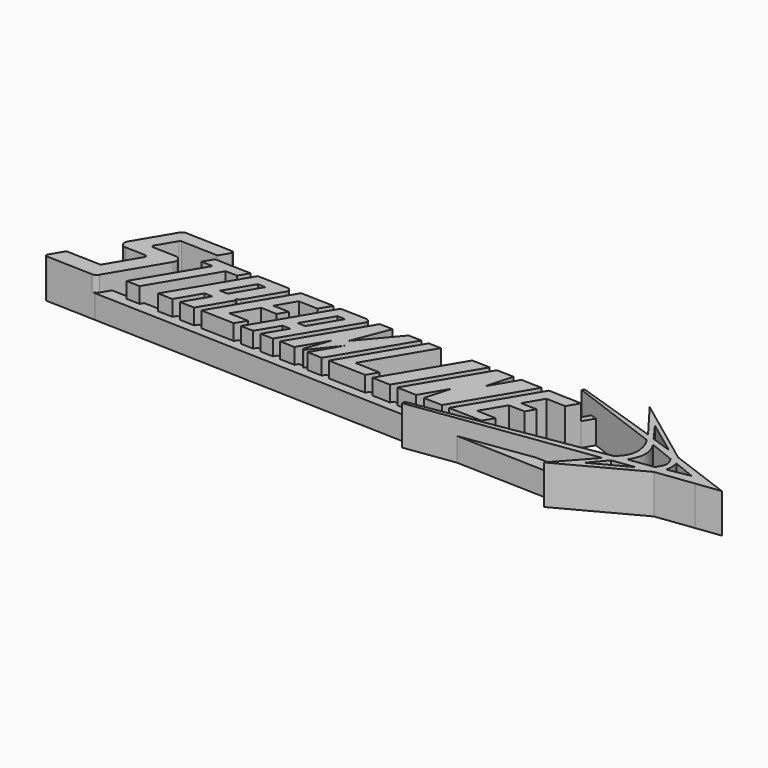
from build123d import *

# Parameters (mm, degrees)
F3_DEPTH    = 5
F4_DEPTH    = 3
F5_DEPTH    = 5
F6_T1_DEPTH = 4.2430941222
F7_R        = 0.75
F8_R        = 0.25
F9_R        = 0.5


# Not quite as in the source:
# - a fillet or chamfer that OpenCascade refuses, or shapes differently, is made with other operations: its cross-section is extruded or revolved along the edge and cut away or added
# - the dataset's text gives a spline's control points without its knots; the knots are read off the source's solid


with BuildPart() as f3:
    # F1 (on Top) → F3 (new body)
    with BuildSketch(Plane.XY):
        with BuildLine():
            Line((20.9890730849, 6.6955136709), (20.8262177718, 6.4128558685))
            Line((20.8262177718, 6.4128558685), (32.5976700121, 2.0520742269))
            add(Edge.make_bspline(
                [(32.5976700121, 2.0520742269), (32.66479791, 1.9612326634), (32.9078702036, 1.6322940043), (33.2495684632, 0.8503160257), (33.5175624456, -0.3144692674), (33.2543808955, -1.5649575024), (32.6660823722, -2.3242091008), (32.2798649798, -2.631161677), (32.1629690369, -2.724066847)],
                knots=[0, 0, 0, 0, 0.338377, 1.225264, 2.537513, 3.868989, 4.900887, 5.348773, 5.348773, 5.348773, 5.348773], degree=3))
            Line((32.1629690369, -2.724066847), (8.6369270261, -6.5884035475))
            Line((8.6369270261, -6.5884035475), (8.6392750964, -6.9738253951))
            Line((8.6392750964, -6.9738253951), (31.5857229554, -3.7504750461))
            Line((31.5857229554, -3.7504750461), (27.6476915727, -8.1477057948))
            Line((27.6476915727, -8.1477057948), (37.4754122714, -2.8992304066))
            Line((37.4754122714, -2.8992304066), (42.2447667452, -2.2940801703))
            Line((42.2447667452, -2.2940801703), (45.3573419295, -1.8991471414))
            Line((45.3573419295, -1.8991471414), (42.1900098482, -0.7209429398))
            Line((42.1900098482, -0.7209429398), (37.4064079021, 1.0584915391))
            Line((37.4064079021, 1.0584915391), (28.4184888939, 7.7636854948))
            Line((28.4184888939, 7.7636854948), (31.9932630947, 3.0268066577))
            Line((31.9932630947, 3.0268066577), (20.9890730849, 6.6955136709))
        make_face()
        Polygon((35.4575661162, -3.2228435634), (30.8492315292, -5.6525000589), (32.5873011966, -3.610950146), align=None, mode=Mode.SUBTRACT)
        with BuildLine():
            Line((36.9164326126, -2.0131677576), (33.7172948492, -2.4477515814))
            add(Edge.make_bspline(
                [(33.7522917412, 1.6292004342), (33.8151917165, 1.5224178068), (34.0236807852, 1.1684709092), (34.316701025, 0.4779029509), (34.496667936, -0.4792529836), (34.2653350207, -1.3976559433), (33.9756190313, -2.0377855614), (33.7761823537, -2.3542949446), (33.7172948492, -2.4477515814)],
                knots=[0, 0, 0, 0, 0.371596, 1.231709, 2.243752, 3.225396, 4.015779, 4.346939, 4.346939, 4.346939, 4.346939], degree=3))
            Line((33.7522917412, 1.6292004342), (37.0218462303, 0.3297472202))
            add(Edge.make_bspline(
                [(36.9164326126, -2.0131677576), (36.9641091848, -1.9397738205), (37.1152370901, -1.7071284219), (37.3297565887, -1.2919332808), (37.4856453978, -0.739306923), (37.33186312, -0.2383098734), (37.1684320619, 0.1026463975), (37.0557106146, 0.2772826387), (37.0218462303, 0.3297472202)],
                knots=[0, 0, 0, 0, 0.262319, 0.831507, 1.406816, 1.920771, 2.356545, 2.543685, 2.543685, 2.543685, 2.543685], degree=3))
        make_face(mode=Mode.SUBTRACT)
        with BuildLine():
            add(Edge.make_bspline(
                [(38.1416125443, -1.7388595712), (38.1499505224, -1.6861617751), (38.1779707155, -1.5090687116), (38.2120498589, -1.1831309562), (38.2229188343, -0.7827452769), (38.1747484177, -0.4294012981), (38.1198989231, -0.1979742905), (38.0817402166, -0.0923088934), (38.0715592092, -0.0641174199)],
                knots=[0, 0, 0, 0, 0.160044, 0.537838, 0.982775, 1.357504, 1.604535, 1.694427, 1.694427, 1.694427, 1.694427], degree=3))
            Line((38.0715592092, -0.0641174199), (40.9662755038, -1.2324347209))
            Line((40.9662755038, -1.2324347209), (38.1416125443, -1.7388595712))
        make_face(mode=Mode.SUBTRACT)
        Polygon((33.0280173393, 2.632852847), (31.3381946618, 4.9499999378), (35.6817278033, 1.7299066189), align=None, mode=Mode.SUBTRACT)
    extrude(amount=F3_DEPTH)

    # F2 (on Top) → F4 (join)
    with BuildSketch(Plane.XY):
        Polygon((30.4451698308, -5.0240238787), (-31.5077020799, -3.0337495602), (-32.4236048399, -4.5718295186), (29.0806183264, -6.5476907188), align=None)
        Polygon((21.6650361648, 4.1573069305), (22.5942029424, 4.1285426611), (23.3891042563, 5.4634243028), (22.6138332811, 5.7506265415), align=None)
    extrude(amount=F4_DEPTH)

    # F0 (on Top) → F5 (join)
    with BuildSketch(Plane.XY):
        Polygon((-37.9180402346, -2.274961737), (-39.1569778781, -4.3555157462), (-32.4236048399, -4.5718295186), (-27.5283611438, 3.6487770236), (-32.0936571446, 3.7954399806), (-30.4533826172, 6.5499609703), (-25.6068335268, 6.4052671518), (-24.6373546626, 8.0333177225), (-31.447669093, 8.2521032848), (-35.1129866215, 2.0969177364), (-30.8469119008, 1.959867448), (-33.4540838572, -2.4183690959), align=None)
        Polygon((-24.5548592656, 4.3197505292), (-29.241506667, -3.5505592413), (-27.5305965593, -3.603523984), (-22.8439491578, 4.2667857865), (-21.3778178633, 4.2213986756), (-20.6361838773, 5.4668282346), (-25.2816460752, 5.6106380753), (-26.0232800612, 4.3652085163), align=None)
        Polygon((-19.6843868267, 5.4373633985), (-25.1126682142, -3.678375931), (-23.2585706727, -3.7357733353), (-21.4998541289, -0.7823520914), (-20.5003329545, -0.813294326), (-22.2590494983, -3.7667155698), (-20.4049519568, -3.8241129742), (-18.1906397432, -0.1056077066), (-18.2790053405, 0.2246448923), (-17.9465448288, 0.3043020701), (-14.9766705694, 5.2916263553), align=None)
        Polygon((-19.6658987552, 0.5879750825), (-20.6654199296, 0.618917317), (-18.6048277351, 4.079279809), (-17.6053065607, 4.0483375745), align=None, mode=Mode.SUBTRACT)
        Polygon((-14.0248735187, 5.2621615192), (-19.4531549062, -3.8535778103), (-15.2273445, -3.9843964663), (-14.4499043415, -2.6788374278), (-16.8926357379, -2.6032176514), (-15.1597178798, 0.3068797341), (-13.124337221, 0.2438703379), (-12.462449258, 1.3553820125), (-14.4978299169, 1.4183914088), (-13.1139875282, 3.7422846611), (-10.6712561318, 3.6666648846), (-9.7990631125, 5.1313428632), align=None)
        Polygon((-8.8472660619, 5.1018780271), (-14.2755474493, -4.0138613024), (-12.6938236683, -4.0628268165), (-11.0875957807, -1.3654805144), (-10.0880746062, -1.3964227489), (-11.6943024939, -4.0937690511), (-10.1125787128, -4.1427345652), (-4.6842973253, 4.9730047642), align=None)
        Polygon((-7.1001108599, 3.6212792995), (-9.2695420463, -0.0218570409), (-10.2690632207, 0.0090851937), (-8.0996320343, 3.652221534), align=None, mode=Mode.SUBTRACT)
        Polygon((-3.7325002747, 4.9435399282), (-9.1607816622, -4.1721994013), (-7.2979875585, -4.2298660256), (-5.2388499842, -0.7719462844), (-6.6666225437, -4.7500652122), (-3.5448452498, -0.8594919276), (-5.5834571721, -4.2829428415), (-3.7206630683, -4.3406094658), (1.7076183191, 4.7751298637), (0.0377097259, 4.8268253201), (-3.8948562166, 0.1842124962), (-2.0625916814, 4.8918444717), align=None)
        Polygon((2.6594153698, 4.7456650276), (-2.7688660177, -4.3700743019), (1.962548568, -4.5165449756), (2.7399887264, -3.2109859371), (-0.4097020782, -3.1134807776), (4.2411391508, 4.6966995134), align=None)
        Polygon((8.3426270061, 4.5697295178), (2.9143456186, -4.5460098117), (5.2055925183, -4.6169400739), (10.6338739058, 4.4987992556), align=None)
        Polygon((11.5856709564, 4.4693344195), (6.157389569, -4.6464049099), (8.6202308493, -4.7226472292), (10.5479239521, -1.4854628282), (9.6247480336, -4.7537441255), (11.9883140981, -4.8269131763), (17.4165954855, 4.2888261532), (14.789173759, 4.3701633988), (12.8065030462, 1.04065483), (13.7560078474, 4.4021471754), align=None)
        Polygon((18.3683925362, 4.2593613171), (12.9401111487, -4.8563780124), (17.1659215549, -4.9871966684), (17.9433617134, -3.6816376299), (15.500630317, -3.6060178535), (17.2335481751, -0.695920468), (19.2689288339, -0.7589298642), (19.9308167969, 0.3525818104), (17.895436138, 0.4155912067), (19.2792785267, 2.739484459), (21.7220099231, 2.6638646825), (22.5942029424, 4.1285426611), align=None)
    extrude(amount=F5_DEPTH)

    # F6: fillet of radius 0.15 on 1 edges, made by hand

    # F6_s2 → F6_t1 (cut)
    with BuildSketch(Plane.XY.offset(3)):
        with BuildLine():
            ThreePointArc((-6.1047892425, -4.0505091099), (-6.2957535157, -4.0876516681), (-6.3639048821, -3.9054366453))
            Line((-6.3639048821, -3.9054366453), (-6.3780745043, -3.9003510764))
            ThreePointArc((-6.3780745043, -3.9003510764), (-6.5292450922, -4.3227329215), (-6.680792166, -4.7449796433))
            Line((-6.680792166, -4.7449796433), (-6.654880602, -4.7594868897))
            ThreePointArc((-6.654880602, -4.7594868897), (-6.3741199427, -4.4095836719), (-6.0930473007, -4.0599307875))
            Line((-6.0930473007, -4.0599307875), (-6.1047892425, -4.0505091099))
        make_face()
    extrude(amount=F6_T1_DEPTH, mode=Mode.SUBTRACT)

    # F7
    f7_edges = [f3.edges().sort_by_distance(p)[0] for p in [
        (-32.423605, -4.57183, 4),
        (-27.528361, 3.648777, 2.5),
        (-35.112987, 2.096918, 2.5),
        (-31.447669, 8.252103, 2.5),
    ]]
    fillet(f7_edges, radius=F7_R)

    # F8
    f8_edges = [f3.edges().sort_by_distance(p)[0] for p in [
        (-25.606834, 6.405267, 2.5),
        (-24.637355, 8.033318, 2.5),
        (-32.093657, 3.79544, 2.5),
        (-30.846912, 1.959867, 2.5),
        (-33.454084, -2.418369, 2.5),
        (-37.91804, -2.274962, 2.5),
        (-39.156978, -4.355516, 2.5),
        (-30.453383, 6.549961, 2.5),
    ]]
    fillet(f8_edges, radius=F8_R)

    # F9
    f9_edges = [f3.edges().sort_by_distance(p)[0] for p in [
        (-14.976671, 5.291626, 2.5),
        (-8.847266, 5.101878, 2.5),
        (-4.684297, 4.973005, 2.5),
        (-17.946545, 0.304302, 2.5),
        (-18.19064, -0.105608, 2.5),
    ]]
    fillet(f9_edges, radius=F9_R)


solid = f3.part
